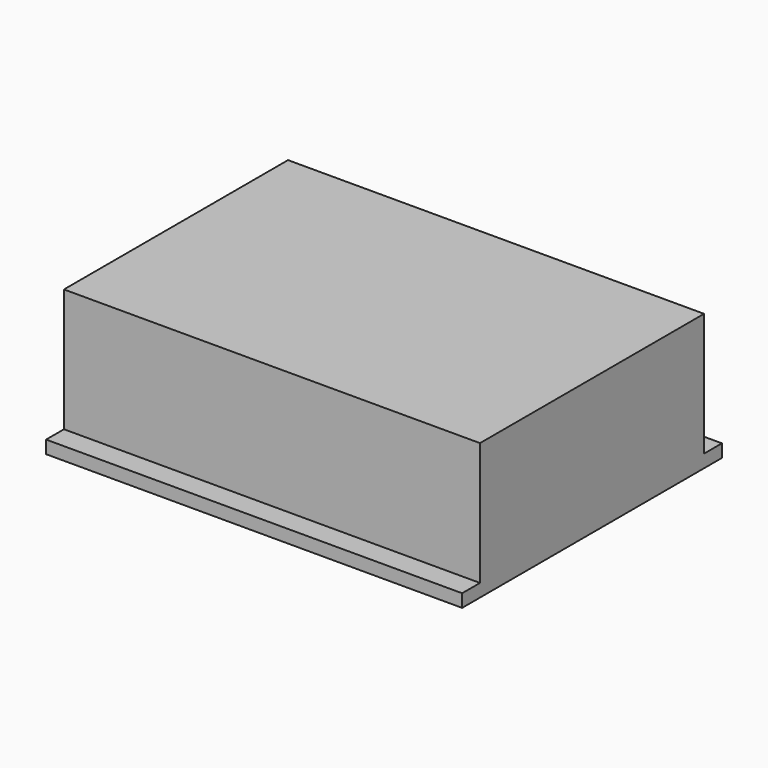
from build123d import *

# Parameters (mm, degrees)
F0_W     = 205
F0_H     = 138
F1_DEPTH = 67
F2_W     = 205
F2_H     = 6.35
F3_DEPTH = 11


# Not quite as in the source:
# - a pattern or mirror of a feature is missing from the dataset's text; its kind, count and spacing are read off the source's solid


with BuildPart() as f1:
    # F0 (on Top) → F1 (new body)
    with BuildSketch(Plane.XY):
        Rectangle(F0_W, F0_H)
    extrude(amount=F1_DEPTH)

    # F2 (on face) → F3 (join)
    with BuildSketch(Plane.XZ.offset(69)):
        with Locations((0, 3.175)):
            Rectangle(F2_W, F2_H)
    f3 = extrude(amount=F3_DEPTH)

    # F3_copies: F3 across plane
    add(f3.mirror(Plane.ZX))


solid = f1.part
